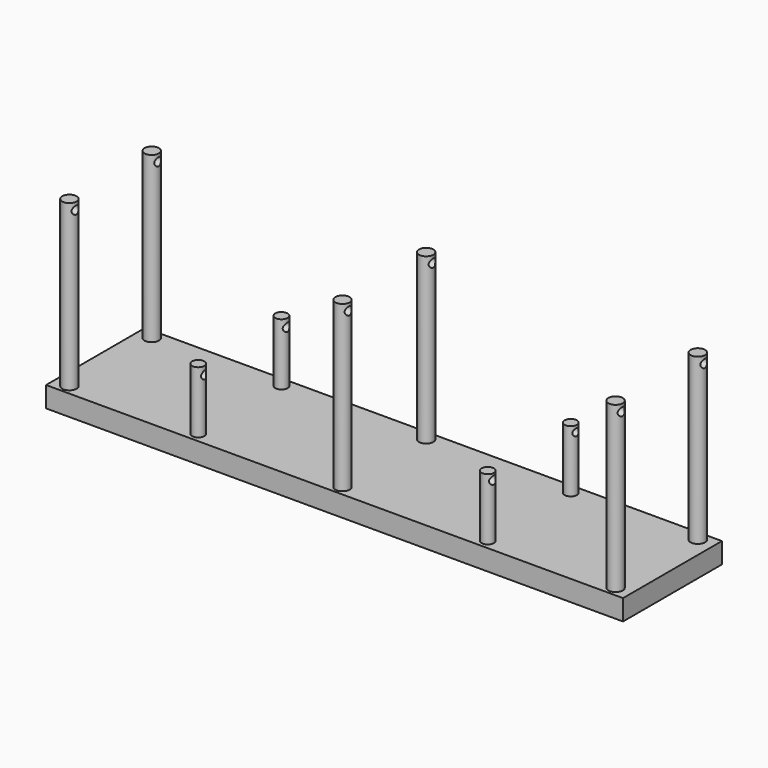
from build123d import *

# Parameters (mm, degrees)
F0_W           = 177.8
F0_H           = 38.1
F1_DEPTH       = 6.35
F3_R           = 2.2225
F4_DEPTH       = 50.8
F5_R           = 1.905
F6_DEPTH       = 19.05
F8_R           = 1.27
F9_DEPTH       = 88.8510297153
F9_DEPTH_BACK  = 88.9509702847
F11_R          = 1.27
F11_R_2        = 1.1088597931
F12_DEPTH      = 25.4
F12_DEPTH_BACK = 25.4
F14_R          = 1.2677185846
F14_R_2        = 1.27
F15_DEPTH      = 25.4
F15_DEPTH_BACK = 25.4


with BuildPart() as f1:
    # F0 (on Top) → F1 (new body)
    with BuildSketch(Plane.XY):
        with Locations((-8.9399702847, -13.2571834021)):
            Rectangle(F0_W, F0_H)
    extrude(amount=F1_DEPTH)

    # F3 (on face) → F4 (join)
    with BuildSketch(Plane.XY.offset(6.35)):
        with Locations((-8.7318996609, 2.7132803676)):
            Circle(F3_R)
        with Locations((-8.9399702847, -29.2450338602)):
            Circle(F3_R)
        with Locations((-93.2964851438, 2.7132803676)):
            Circle(F3_R)
        with Locations((-93.08841452, -29.2450338602)):
            Circle(F3_R)
        with Locations((75.0004033269, 2.7132803676)):
            Circle(F3_R)
        with Locations((75.2084739506, -29.2450338602)):
            Circle(F3_R)
    extrude(amount=F4_DEPTH)

    # F5 (on face) → F6 (join)
    with BuildSketch(Plane.XY.offset(6.35)):
        with Locations((-53.323045761, 2.7132803676)):
            Circle(F5_R)
        with Locations((-53.3533677751, -29.3119172592)):
            Circle(F5_R)
        with Locations((35.8592464392, 2.7132803676)):
            Circle(F5_R)
        with Locations((35.8895684532, -29.3119172592)):
            Circle(F5_R)
    extrude(amount=F6_DEPTH)

    # F8 (on offset) → F9 (cut, two sides)
    with BuildSketch(Plane.YZ.offset(-8.89)) as f9_sk:
        with Locations((2.6895276339, 54.9170612506)):
            Circle(F8_R)
        with Locations((-29.3519098263, 54.9170612506)):
            Circle(F8_R)
    extrude(amount=F9_DEPTH, mode=Mode.SUBTRACT)
    extrude(f9_sk.sketch, amount=-F9_DEPTH_BACK, mode=Mode.SUBTRACT)

    # F11 (on offset) → F12 (cut, two sides)
    with BuildSketch(Plane.YZ.offset(35.56)) as f12_sk:
        with Locations((-29.3395008357, 23.487156257)):
            Circle(F11_R)
        with Locations((2.5792657398, 23.487156257)):
            Circle(F11_R_2)
    extrude(amount=-F12_DEPTH, mode=Mode.SUBTRACT)
    extrude(f12_sk.sketch, amount=F12_DEPTH_BACK, mode=Mode.SUBTRACT)

    # F14 (on offset) → F15 (cut, two sides)
    with BuildSketch(Plane.YZ.offset(-53.34)) as f15_sk:
        with Locations((2.7075121179, 22.8937678039)):
            Circle(F14_R)
        with Locations((-29.0134996176, 22.8937678039)):
            Circle(F14_R_2)
    extrude(amount=-F15_DEPTH, mode=Mode.SUBTRACT)
    extrude(f15_sk.sketch, amount=F15_DEPTH_BACK, mode=Mode.SUBTRACT)


solid = f1.part
